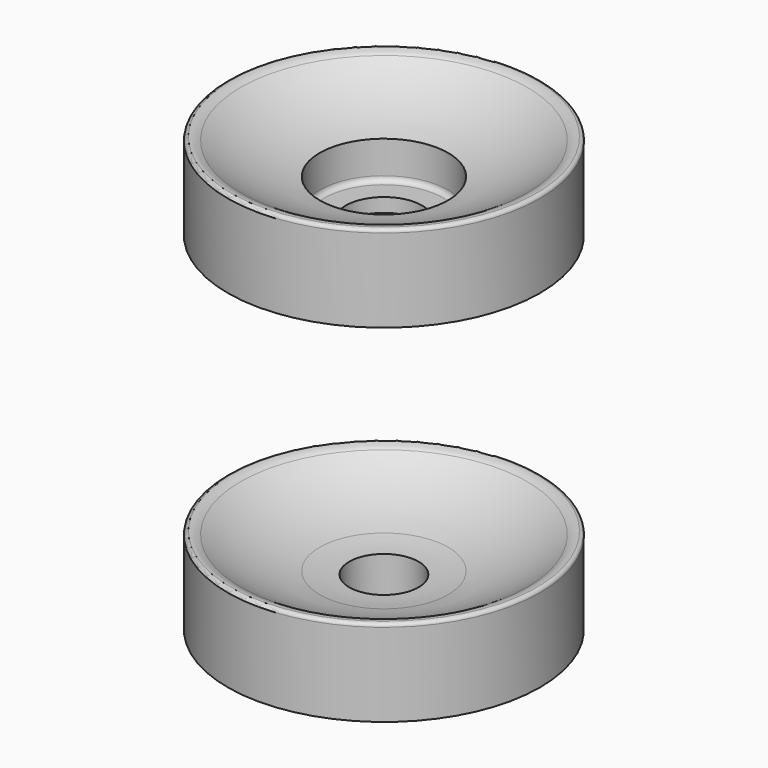
from build123d import *

# Parameters (mm, degrees)
F0_W = 0.2
F0_H = 0.8


# Not quite as in the source:
# - ends of sketch curves that miss each other by under 0.0002 mm in the source are joined


with BuildPart() as f1:
    # F0 (on Front) → F1 (revolve)
    with BuildSketch(Plane.XZ):
        with BuildLine():
            Line((-3.7, 1.1), (-3.7, 2.9801763189))
            ThreePointArc((-3.7, 2.9801763189), (-6.0731435, 3.6667135458), (-8.2532045739, 4.8288138641))
            ThreePointArc((-8.2532045739, 4.8288138641), (-8.514086333, 4.9543650035), (-8.8000010311, 4.9999189962))
            ThreePointArc((-8.8000010311, 4.9999189962), (-8.9414213562, 4.9414213562), (-9, 4.8))
            Line((-9, 4.8), (-9, 0))
            Line((-9, 0), (-8.2, 0))
            Line((-8.2, 0), (-8.2, 2))
            Line((-8.2, 2), (-6, 2))
            Line((-6, 2), (-4, 0))
            Line((-4, 0), (-2.2, 0))
            Line((-2.2, 0), (-2.2, 0.8))
            Line((-2.2, 0.8), (-3.4, 0.8))
            ThreePointArc((-3.4, 0.8), (-3.6121320344, 0.8878679656), (-3.7, 1.1))
        make_face()
        with Locations((-2.1, 0.4)):
            Rectangle(F0_W, F0_H)
        with BuildLine():
            Line((-2, 0.8), (-2, 2.8))
            ThreePointArc((-2, 2.8), (-2.853242146, 2.8594978565), (-3.7, 2.9801763189))
            Line((-3.7, 2.9801763189), (-3.7, 1.1))
            ThreePointArc((-3.7, 1.1), (-3.6121320344, 0.8878679656), (-3.4, 0.8))
            Line((-3.4, 0.8), (-2.2, 0.8))
            Line((-2.2, 0.8), (-2, 0.8))
        make_face()
    revolve(axis=Axis((0, 0, 1.133464626), (0, 0, 1)))


with BuildPart() as f1_1:
    # F2: moved
    add(f1.part.moved(Location((0, 0, -20))))


with BuildPart() as f3:
    # F0 (on Front) → F3 (revolve)
    with BuildSketch(Plane.XZ):
        with BuildLine():
            Line((-3.7, 1.1), (-3.7, 2.9801763189))
            ThreePointArc((-3.7, 2.9801763189), (-6.0731435, 3.6667135458), (-8.2532045739, 4.8288138641))
            ThreePointArc((-8.2532045739, 4.8288138641), (-8.514086333, 4.9543650035), (-8.8000010311, 4.9999189962))
            ThreePointArc((-8.8000010311, 4.9999189962), (-8.9414213562, 4.9414213562), (-9, 4.8))
            Line((-9, 4.8), (-9, 0))
            Line((-9, 0), (-8.2, 0))
            Line((-8.2, 0), (-8.2, 2))
            Line((-8.2, 2), (-6, 2))
            Line((-6, 2), (-4, 0))
            Line((-4, 0), (-2.2, 0))
            Line((-2.2, 0), (-2.2, 0.8))
            Line((-2.2, 0.8), (-3.4, 0.8))
            ThreePointArc((-3.4, 0.8), (-3.6121320344, 0.8878679656), (-3.7, 1.1))
        make_face()
    revolve(axis=Axis((0, 0, 1.133464626), (0, 0, 1)))


solid = Compound([f1_1.part, f3.part])
